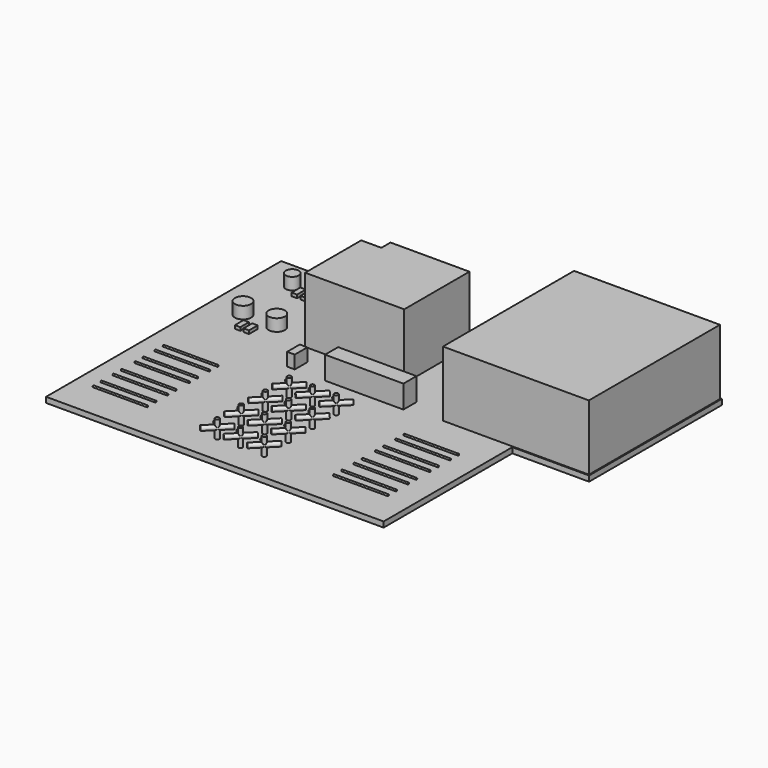
from build123d import *

# Parameters (mm, degrees)
F0_W      = 4700
F0_H      = 2000
F1_DEPTH  = 500
F2_W      = 13400
F2_H      = 15050
F3_DEPTH  = 6000
F5_DEPTH  = 6000
F6_W      = 7200
F6_H      = 1500
F7_DEPTH  = 2100
F8_R      = 600
F9_DEPTH  = 1100
F8_R_2    = 750
F10_W     = 500
F10_H     = 1000
F11_DEPTH = 300
F12_R     = 190.5
F13_DEPTH = 1615
F14_R     = 209.5
F15_DEPTH = 2458
F16_ANGLE = 90
F20_ANGLE = 45
F21_R     = 207
F22_DEPTH = 955
F23_ANGLE = 90
F25_ANGLE = 315
F36_R     = 75
F37_DEPTH = 5000
F38_ANGLE = 90
F40_ANGLE = 90
F46_W     = 1500
F46_H     = 3000
F47_DEPTH = 1200
F46_W_2   = 700
F46_H_2   = 1450


with BuildPart() as f1:
    # F0 (on Top) → F1 (new body)
    with BuildSketch(Plane.XY):
        Polygon((0, 26990), (0, 0), (31000, 0), (31000, 14775), (38050, 14775), (38050, 30025), (24450, 30025), (24450, 26990), (9300, 26990), (4600, 26990), align=None)
        with Locations((6950, 27990)):
            Rectangle(F0_W, F0_H)
    extrude(amount=F1_DEPTH)


with BuildPart() as f3:
    # F2 (on face) → F3 (new body)
    with BuildSketch(Plane.XY.offset(500)):
        with Locations((31250, 22400)):
            Rectangle(F2_W, F2_H)
    extrude(amount=F3_DEPTH)


with BuildPart() as f5:
    # F4 (on face) → F5 (new body)
    with BuildSketch(Plane.XY.offset(500)):
        Polygon((11520, 24090), (9670, 24090), (9670, 17655), (18770, 17655), (18770, 25140), (11520, 25140), align=None)
    extrude(amount=F5_DEPTH)


with BuildPart() as f7:
    # F6 (on face) → F7 (new body)
    with BuildSketch(Plane.XY.offset(500)):
        with Locations((17654, 15205)):
            Rectangle(F6_W, F6_H)
    extrude(amount=F7_DEPTH)


with BuildPart() as f9:
    # F8 (on face) → F9 (new body)
    with BuildSketch(Plane.XY.offset(500)):
        with Locations((3100, 24390)):
            Circle(F8_R)
    extrude(amount=F9_DEPTH)


with BuildPart() as f9b:
    # F8 (on face) → F9, piece 2 (new body)
    with BuildSketch(Plane.XY.offset(500)):
        with Locations((6200, 24390)):
            Circle(F8_R)
    extrude(amount=F9_DEPTH)


with BuildPart() as f9c:
    # F8 (on face) → F9, piece 3 (new body)
    with BuildSketch(Plane.XY.offset(500)):
        with Locations((3055.5453419685, 18790)):
            Circle(F8_R_2)
    extrude(amount=F9_DEPTH)


with BuildPart() as f9d:
    # F8 (on face) → F9, piece 4 (new body)
    with BuildSketch(Plane.XY.offset(500)):
        with Locations((6155.5453419685, 18790)):
            Circle(F8_R_2)
    extrude(amount=F9_DEPTH)


with BuildPart() as f11:
    # F10 (on face) → F11 (new body)
    with BuildSketch(Plane.XY.offset(500)):
        with Locations((4250, 23690)):
            Rectangle(F10_W, F10_H)
    extrude(amount=F11_DEPTH)


with BuildPart() as f11b:
    # F10 (on face) → F11, piece 2 (new body)
    with BuildSketch(Plane.XY.offset(500)):
        with Locations((5050, 23690)):
            Rectangle(F10_W, F10_H)
    extrude(amount=F11_DEPTH)


with BuildPart() as f11c:
    # F10 (on face) → F11, piece 3 (new body)
    with BuildSketch(Plane.XY.offset(500)):
        with Locations((4230.5389404297, 17194.1223144531)):
            Rectangle(F10_W, F10_H)
    extrude(amount=F11_DEPTH)


with BuildPart() as f11d:
    # F10 (on face) → F11, piece 4 (new body)
    with BuildSketch(Plane.XY.offset(500)):
        with Locations((5030.5389404297, 17194.1223144531)):
            Rectangle(F10_W, F10_H)
    extrude(amount=F11_DEPTH)


with BuildPart() as f13:
    # F12 (on face) → F13 (new body)
    with BuildSketch(Plane.XY.offset(500)):
        with Locations((13620, 2628)):
            Circle(F12_R)
    extrude(amount=F13_DEPTH)


with BuildPart() as f15:
    # F14 (on face) → F15 (new body)
    with BuildSketch(Plane.XY.offset(500)):
        with Locations((15123.7049102783, 3486.6054058075)):
            Circle(F14_R)
    extrude(amount=F15_DEPTH)


with BuildPart() as f15_1:
    # F16: moved
    add(f15.part.rotate(Axis((15500, 0, 500), (1, 0, 0)), F16_ANGLE))


with BuildPart() as f15_2:
    # F17: moved
    add(f15_1.part.moved(Location((-1510, 3860, -2600))))


with BuildPart() as f15_3:
    # F18: moved
    add(f15_2.part.moved(Location((0, 0, 939))))


with BuildPart() as f15_4:
    # F19: moved
    add(f15_3.part.moved(Location((0, 0, -930))))


with BuildPart() as f15_5:
    # F20: moved
    add(f15_4.part.rotate(Axis((13620, 2628, 500), (0, 0, -1)), F20_ANGLE))


with BuildPart() as f22:
    # F21 (on face) → F22 (new body)
    with BuildSketch(Plane.XY.offset(500)):
        with Locations((10922.384262085, 1929.0287494659)):
            Circle(F21_R)
    extrude(amount=F22_DEPTH)


with BuildPart() as f22_1:
    # F23: moved
    add(f22.part.rotate(Axis((15500, 0, 500), (1, 0, 0)), F23_ANGLE))


with BuildPart() as f22_2:
    # F24: moved
    add(f22_1.part.moved(Location((2700, 3450, -1023))))


with BuildPart() as f22_3:
    # F25: moved
    add(f22_2.part.rotate(Axis((13620, 2628, 500), (0, 0, -1)), F25_ANGLE))


with BuildPart() as f15_6:
    add(f15_5.part)

    # F26: union F22, F13
    add(f22_3.part)
    add(f13.part)


with BuildPart() as f28_1:
    # F28: copy of F15
    add(f15_6.part)


with BuildPart() as f29_1:
    # F29: copy of F15
    add(f15_6.part.moved(Location((1882, 0, 0))))


with BuildPart() as f29_2:
    # F29: copy of F28_1
    add(f28_1.part.moved(Location((1882, 0, 0))))


with BuildPart() as f30_1:
    # F30: copy of F29_1
    add(f29_1.part.moved(Location((2436, 0, 0))))


with BuildPart() as f30_2:
    # F30: copy of F29_2
    add(f29_2.part.moved(Location((2436, 0, 0))))


with BuildPart() as f29_1_1:
    # F31: moved
    add(f29_1.part.moved(Location((260, 0, 0))))


with BuildPart() as f29_2_1:
    # F31: moved
    add(f29_2.part.moved(Location((260, 0, 0))))


with BuildPart() as f33_1:
    # F33: copy of F15
    add(f15_6.part.moved(Location((0, 2760, 0))))


with BuildPart() as f33_2:
    # F33: copy of F29_1
    add(f29_1_1.part.moved(Location((0, 2760, 0))))


with BuildPart() as f33_3:
    # F33: copy of F30_1
    add(f30_1.part.moved(Location((0, 2760, 0))))


with BuildPart() as f33_4:
    # F33: copy of F29_2
    add(f29_2_1.part.moved(Location((0, 2760, 0))))


with BuildPart() as f33_5:
    # F33: copy of F30_2
    add(f30_2.part.moved(Location((0, 2760, 0))))


with BuildPart() as f33_6:
    # F33: copy of F28_1
    add(f28_1.part.moved(Location((0, 2760, 0))))


with BuildPart() as f34_1:
    # F34: copy of F33_1
    add(f33_1.part.moved(Location((0, 2760, 0))))


with BuildPart() as f34_2:
    # F34: copy of F33_2
    add(f33_2.part.moved(Location((0, 2760, 0))))


with BuildPart() as f34_3:
    # F34: copy of F33_3
    add(f33_3.part.moved(Location((0, 2760, 0))))


with BuildPart() as f34_4:
    # F34: copy of F33_4
    add(f33_4.part.moved(Location((0, 2760, 0))))


with BuildPart() as f34_5:
    # F34: copy of F33_6
    add(f33_6.part.moved(Location((0, 2760, 0))))


with BuildPart() as f34_6:
    # F34: copy of F33_5
    add(f33_5.part.moved(Location((0, 2760, 0))))


with BuildPart() as f35_1:
    # F35: copy of F34_3
    add(f34_3.part.moved(Location((0, 2740, 0))))


with BuildPart() as f35_2:
    # F35: copy of F34_2
    add(f34_2.part.moved(Location((0, 2740, 0))))


with BuildPart() as f35_3:
    # F35: copy of F34_1
    add(f34_1.part.moved(Location((0, 2740, 0))))


with BuildPart() as f35_4:
    # F35: copy of F34_6
    add(f34_6.part.moved(Location((0, 2740, 0))))


with BuildPart() as f35_5:
    # F35: copy of F34_4
    add(f34_4.part.moved(Location((0, 2740, 0))))


with BuildPart() as f35_6:
    # F35: copy of F34_5
    add(f34_5.part.moved(Location((0, 2740, 0))))


with BuildPart() as f37:
    # F36 (on face) → F37 (new body)
    with BuildSketch(Plane.XY.offset(500)):
        with Locations((2614.0184402466, 3180.5305480957)):
            Circle(F36_R)
    extrude(amount=F37_DEPTH)


with BuildPart() as f37_1:
    # F38: moved
    add(f37.part.rotate(Axis((7750, 0, 500), (1, 0, 0)), F38_ANGLE))


with BuildPart() as f37_2:
    # F39: moved
    add(f37_1.part.moved(Location((0, 5060, -2900))))


with BuildPart() as f37_3:
    # F40: moved
    add(f37_2.part.rotate(Axis((13620, 2628, 500), (0, 0, -1)), F40_ANGLE))


with BuildPart() as f37_4:
    # F41: moved
    add(f37_3.part.moved(Location((-9100, -10670, 0))))


with BuildPart() as f42_1:
    # F42: copy of F37
    add(f37_4.part.moved(Location((0, 940, 0))))


with BuildPart() as f43_1:
    # F43: copy of F37
    add(f37_4.part.moved(Location((0, 2320, 0))))


with BuildPart() as f43_2:
    # F43: copy of F42_1
    add(f42_1.part.moved(Location((0, 2320, 0))))


with BuildPart() as f44_1:
    # F44: copy of F37
    add(f37_4.part.moved(Location((0, 4800, 0))))


with BuildPart() as f44_2:
    # F44: copy of F43_2
    add(f43_2.part.moved(Location((0, 4800, 0))))


with BuildPart() as f44_3:
    # F44: copy of F42_1
    add(f42_1.part.moved(Location((0, 4800, 0))))


with BuildPart() as f44_4:
    # F44: copy of F43_1
    add(f43_1.part.moved(Location((0, 4800, 0))))


with BuildPart() as f45_1:
    # F45: copy of F37
    add(f37_4.part.moved(Location((22100, 0, 0))))


with BuildPart() as f45_2:
    # F45: copy of F43_2
    add(f43_2.part.moved(Location((22100, 0, 0))))


with BuildPart() as f45_3:
    # F45: copy of F44_2
    add(f44_2.part.moved(Location((22100, 0, 0))))


with BuildPart() as f45_4:
    # F45: copy of F44_4
    add(f44_4.part.moved(Location((22100, 0, 0))))


with BuildPart() as f45_5:
    # F45: copy of F42_1
    add(f42_1.part.moved(Location((22100, 0, 0))))


with BuildPart() as f45_6:
    # F45: copy of F43_1
    add(f43_1.part.moved(Location((22100, 0, 0))))


with BuildPart() as f45_7:
    # F45: copy of F44_3
    add(f44_3.part.moved(Location((22100, 0, 0))))


with BuildPart() as f45_8:
    # F45: copy of F44_1
    add(f44_1.part.moved(Location((22100, 0, 0))))


with BuildPart() as f47:
    # F46 (on face) → F47 (new body)
    with BuildSketch(Plane.XY.offset(500)):
        with Locations((20770, 23640)):
            Rectangle(F46_W, F46_H)
    extrude(amount=F47_DEPTH)


with BuildPart() as f47b:
    # F46 (on face) → F47, piece 2 (new body)
    with BuildSketch(Plane.XY.offset(500)):
        with Locations((10924, 15180)):
            Rectangle(F46_W_2, F46_H_2)
    extrude(amount=F47_DEPTH)


solid = Compound([f1.part, f3.part, f5.part, f7.part, f9.part, f9b.part, f9c.part, f9d.part, f11.part, f11b.part, f11c.part, f11d.part, f15_6.part, f28_1.part, f30_1.part, f30_2.part, f29_1_1.part, f29_2_1.part, f33_1.part, f33_2.part, f33_3.part, f33_4.part, f33_5.part, f33_6.part, f34_1.part, f34_2.part, f34_3.part, f34_4.part, f34_5.part, f34_6.part, f35_1.part, f35_2.part, f35_3.part, f35_4.part, f35_5.part, f35_6.part, f37_4.part, f42_1.part, f43_1.part, f43_2.part, f44_1.part, f44_2.part, f44_3.part, f44_4.part, f45_1.part, f45_2.part, f45_3.part, f45_4.part, f45_5.part, f45_6.part, f45_7.part, f45_8.part, f47.part, f47b.part])
